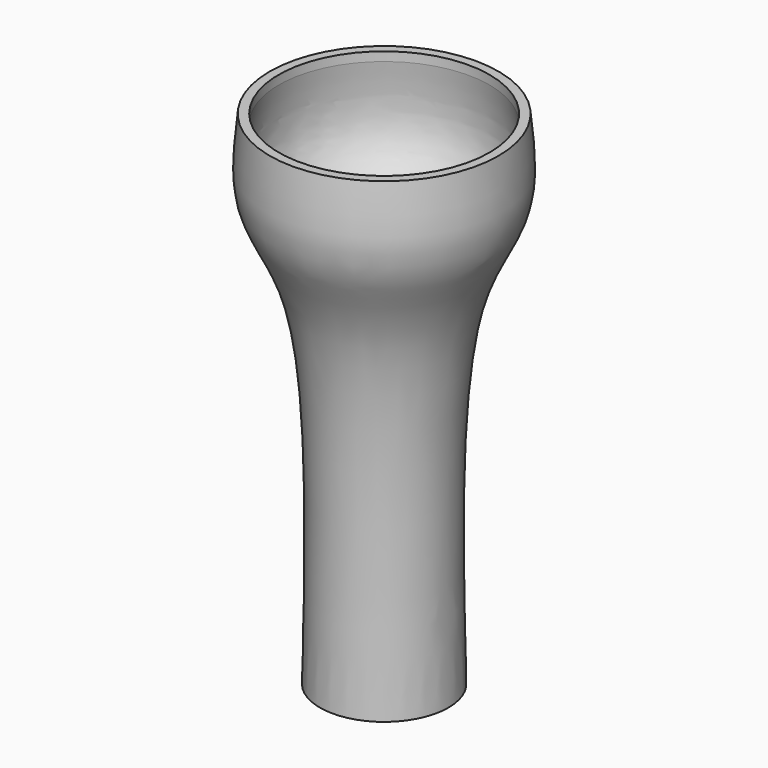
from build123d import *


with BuildPart() as f1:
    # F0 (on Front) → F1 (revolve)
    with BuildSketch(Plane.XZ):
        with BuildLine():
            Line((16.8338194489, 73.9073976874), (15.5150508508, 73.9073976874))
            Line((15.5150508508, 73.9073976874), (15.5150508508, 72.5835412741))
            add(Edge.make_bspline(
                [(15.5150508508, 72.5835412741), (15.9628923537, 69.2326291989), (16.9325939715, 61.9769710258), (6.0200782442, 50.6483344758), (7.3816749001, 20.6485499873), (8.3321169346, 0.7194833016)],
                knots=[0, 0, 0, 0, 0.2241648732, 0.4853794006, 0.9938809288, 0.9938809288, 0.9938809288, 0.9938809288], degree=3))
            add(Edge.make_bspline(
                [(8.3321169346, 0.7194833016), (8.3435541127, 0.4796661682), (8.3549986647, 0.2398330841), (8.3664432168, 0)],
                knots=[0.9938809288, 0.9938809288, 0.9938809288, 0.9938809288, 1, 1, 1, 1], degree=3))
            Line((8.3664432168, 0), (9.4546116889, 0))
            add(Edge.make_bspline(
                [(16.8338194489, 73.9073976874), (17.2893102356, 69.8610769677), (18.2288330573, 61.5148913338), (8.4121151546, 49.9235241023), (9.0389554089, 19.9051273823), (9.4546116889, 0)],
                knots=[0, 0, 0, 0, 0.2407197295, 0.4965230607, 1, 1, 1, 1], degree=3))
        make_face()
        with BuildLine():
            add(Edge.make_bspline(
                [(8.3321169346, 0.7194833016), (8.3435541127, 0.4796661682), (8.3549986647, 0.2398330841), (8.3664432168, 0)],
                knots=[0.9938809288, 0.9938809288, 0.9938809288, 0.9938809288, 1, 1, 1, 1], degree=3))
            Line((8.3321169346, 0.7194833016), (0, 0.7194833016))
            Line((0, 0.7194833016), (0, 0))
            Line((0, 0), (8.3664432168, 0))
        make_face()
    revolve(axis=Axis((0, 0, -9.8443220777), (0, 0, -1)))


solid = f1.part
